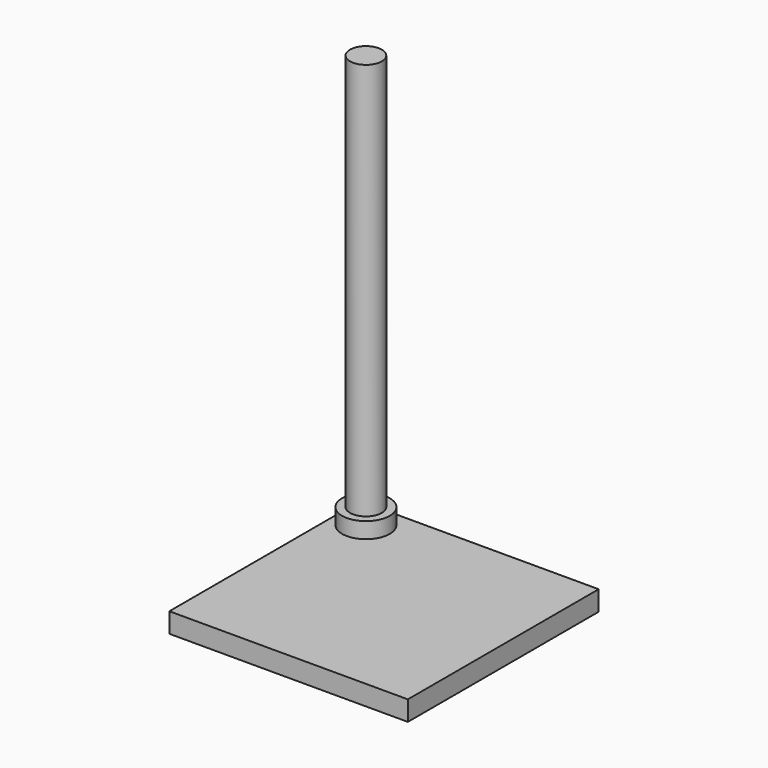
from build123d import *

# Parameters (mm, degrees)
F0_W     = 76.2
F0_H     = 76.2
F0_R     = 7.62
F0_R_2   = 5.08
F1_DEPTH = 6.35
F2_DEPTH = 132.08
F3_DEPTH = 5.08


# Not quite as in the source:
# - a feature names something its author has since deleted; it is built from what else it names


with BuildPart() as f1:
    # F0 (on Top) → F1 (new body)
    with BuildSketch(Plane.XY):
        with Locations((-17.4512108788, -34.2747404939)):
            Rectangle(F0_W, F0_H)
        with Locations((-46.3251647948, -5.4007865778)):
            Circle(F0_R, mode=Mode.SUBTRACT)
        with Locations((-46.3251647948, -5.4007865778)):
            Circle(F0_R)
        with Locations((-46.3251647948, -5.4007865778)):
            Circle(F0_R_2, mode=Mode.SUBTRACT)
        with Locations((-46.3251647948, -5.4007865778)):
            Circle(F0_R_2)
    extrude(amount=-F1_DEPTH)

    # F0 (on Top) → F2 (join)
    with BuildSketch(Plane.XY):
        with Locations((-46.3251647948, -5.4007865778)):
            Circle(F0_R_2)
    extrude(amount=F2_DEPTH)

    # F0 (on Top) → F3 (join)
    with BuildSketch(Plane.XY):
        with Locations((-46.3251647948, -5.4007865778)):
            Circle(F0_R)
        with Locations((-46.3251647948, -5.4007865778)):
            Circle(F0_R_2, mode=Mode.SUBTRACT)
    extrude(amount=F3_DEPTH)


solid = f1.part
